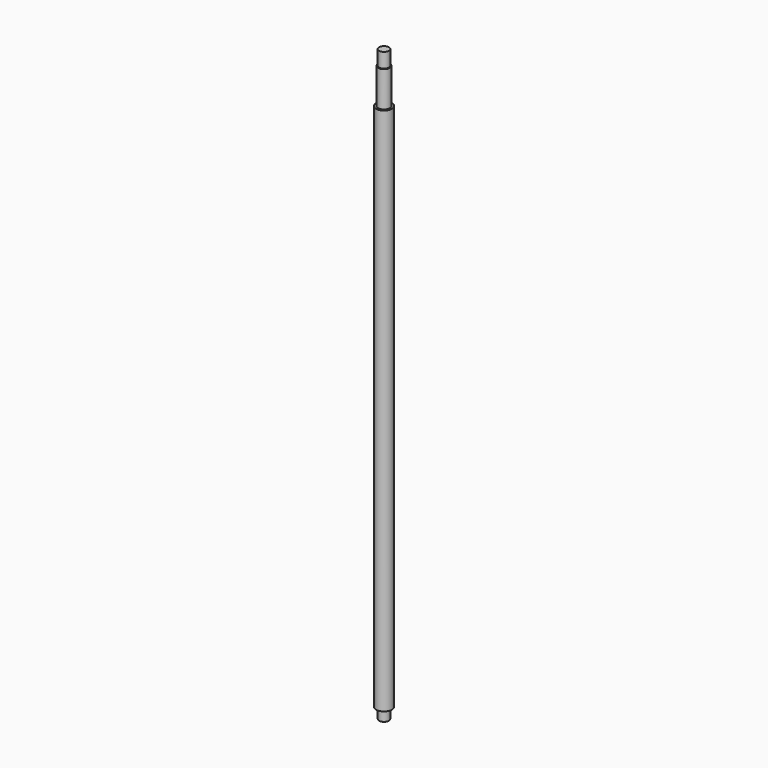
from build123d import *

# Parameters (mm, degrees)
F0_W   = 5
F0_H   = 15
F0_W_2 = 6
F0_H_2 = 22
F0_H_3 = 11
F3_R   = 0.2


# Not quite as in the source:
# - the program builds the solid bodies; features that only make, move or delete a surface that nothing else refers to are left out


with BuildPart() as f1:
    # F0 (on Front) → F1 (revolve)
    with BuildSketch(Plane.XZ):
        with Locations((2.5, 312.5)):
            Rectangle(F0_W, F0_H)
    revolve(axis=Axis((0, 0, -110.3163262457), (0, 0, -1)))



with BuildPart() as f1b:
    # F0 (on Front) → F1, piece 2 (revolve)
    with BuildSketch(Plane.XZ):
        with Locations((3, 280)):
            Rectangle(F0_W_2, F0_H_2)
        Polygon((0, 269), (0, 59.3673475087), (0, -269), (5, -269), (8.025, -269), (8.025, 269), (6, 269), align=None)
        with Locations((2.5, -274.5)):
            Rectangle(F0_W, F0_H_3)
    revolve(axis=Axis((0, 0, -110.3163262457), (0, 0, -1)))


with BuildPart() as f1_1:
    add(f1.part)

    add(f1b.part)  # F2 merges F1b
    # F0 (on Front) → F2 (revolve)
    with BuildSketch(Plane.XZ):
        Polygon((0, 305), (0, 291), (6, 291), (6, 305), (5, 305), align=None)
    revolve(axis=Axis((0, 0, 189.6836737543), (0, 0, 1)))

    # F3
    f3_edges = [f1_1.edges().sort_by_distance(p)[0] for p in [
        (-5, 0, -280),
    ]]
    fillet(f3_edges, radius=F3_R)


solid = f1_1.part
